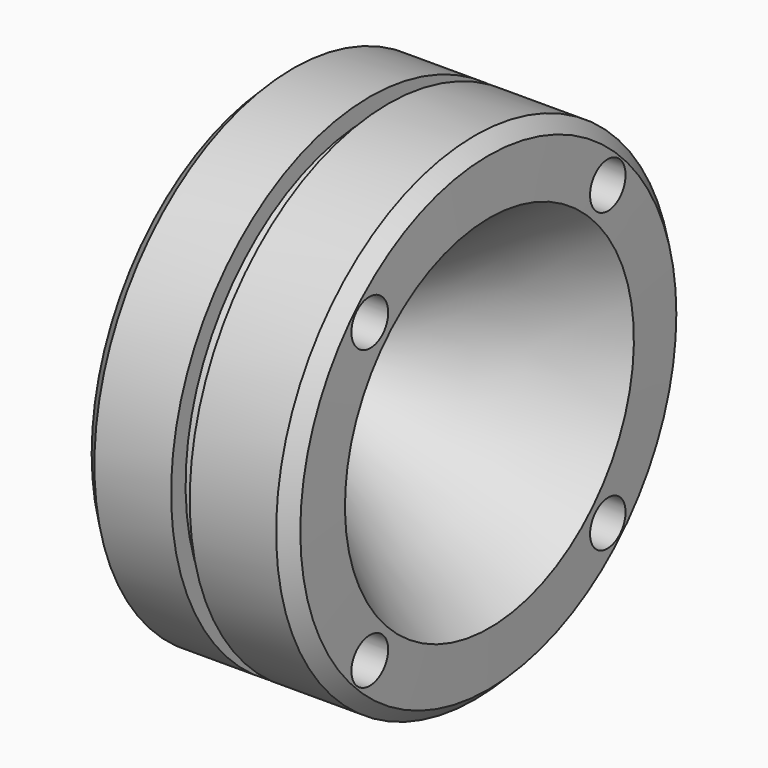
from build123d import *

# Parameters (mm, degrees)
F4_R     = 3.175
F5_DEPTH = 12.7


# Not quite as in the source:
# - a fillet or chamfer that OpenCascade refuses, or shapes differently, is made with other operations: its cross-section is extruded or revolved along the edge and cut away or added


with BuildPart() as f1:
    # F0 (on Front) → F1 (revolve)
    with BuildSketch(Plane.XZ):
        Polygon((0, 7.9375), (5.6608929044, 7.8860616331), (29.5304771808, 25.4019652116), (29.337, 34.925), (15.3162, 34.925), (15.3162, 32.385), (12.7, 32.385), (12.7, 34.925), (0, 34.925), align=None)
    revolve(axis=Axis((10.2213714272, 0, 0), (1, 0, 0)))

    # F2: chamfer of 1.905 on 2 edges, made by hand

    # F2_s1 → F2_t2 (revolve, cut)
    with BuildSketch(Plane.XZ):
        Polygon((1.905, 34.925), (0, 33.02), (0, 34.925), align=None)
    revolve(axis=Axis((0, 0, 0), (1, 0, 0)), mode=Mode.SUBTRACT)

    # F2_s3 → F2_t4 (revolve, cut)
    with BuildSketch(Plane.XZ):
        Polygon((29.3749172557, 33.0586954362), (27.4703102981, 34.925), (29.337, 34.925), align=None)
    revolve(axis=Axis((29.337, 0, 0), (1, 0, 0)), mode=Mode.SUBTRACT)

    # F4 (on offset) → F5 (cut)
    with BuildSketch(Plane.YZ.offset(33.655)):
        with Locations((20.9239967621, 20.9239967621)):
            Circle(F4_R)
        with Locations((20.9239967621, -20.9239967621)):
            Circle(F4_R)
        with Locations((-20.9239967621, -20.9239967621)):
            Circle(F4_R)
        with Locations((-20.9239967621, 20.9239967621)):
            Circle(F4_R)
    extrude(amount=-F5_DEPTH, mode=Mode.SUBTRACT)


solid = f1.part
